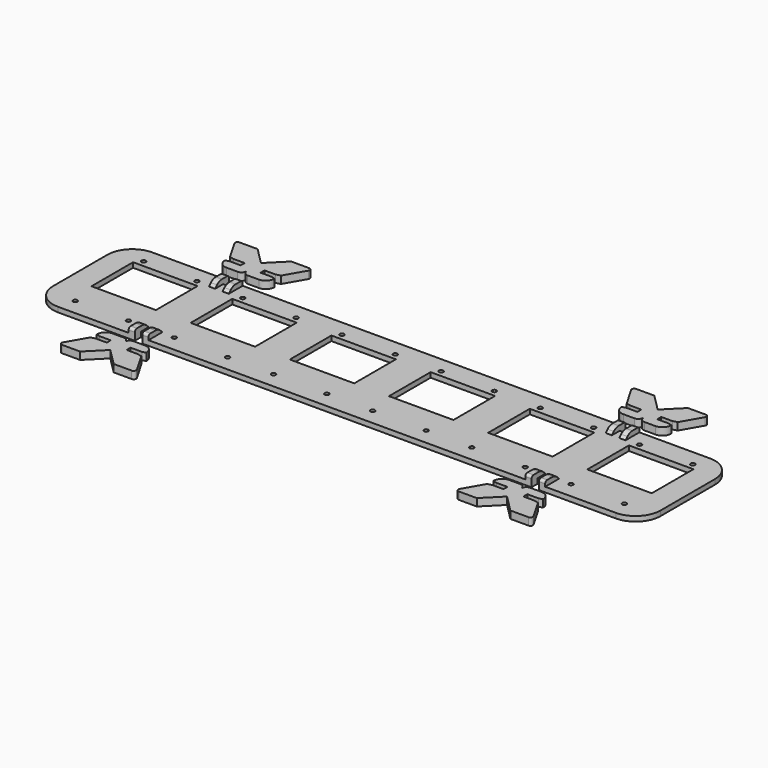
from build123d import *

# Parameters (mm, degrees)
F0_R     = 1.75
F0_W     = 52
F0_H     = 42
F1_DEPTH = 4
F2_R     = 20
F4_DEPTH = 6
F6_DEPTH = 4
F7_SIZE  = 3.99999
F8_R     = 7
F9_R     = 2


# Not quite as in the source:
# - a fillet or chamfer is up to 0.001 mm smaller than in the source, because OpenCascade refuses the exact size


with BuildPart() as f1:
    # F0 (on Top) → F1 (new body)
    with BuildSketch(Plane.XY):
        Polygon((-245, 47.5), (-245, -47.5), (-163, -47.5), (-163, -41.5), (-157, -41.5), (-157, -47.5), (157, -47.5), (157, -41.5), (163, -41.5), (163, -47.5), (245, -47.5), (245, 47.5), (163, 47.5), (163, 41.5), (157, 41.5), (157, 47.5), (-157, 47.5), (-157, 41.5), (-163, 41.5), (-163, 47.5), align=None)
        with Locations((-221.5, -34.5)):
            Circle(F0_R, mode=Mode.SUBTRACT)
        with Locations((-178.5, -34.5)):
            Circle(F0_R, mode=Mode.SUBTRACT)
        with Locations((-141.5, -34.5)):
            Circle(F0_R, mode=Mode.SUBTRACT)
        with Locations((-98.5, -34.5)):
            Circle(F0_R, mode=Mode.SUBTRACT)
        with Locations((-61.5, -34.5)):
            Circle(F0_R, mode=Mode.SUBTRACT)
        with Locations((-18.5, -34.5)):
            Circle(F0_R, mode=Mode.SUBTRACT)
        with Locations((18.5, -34.5)):
            Circle(F0_R, mode=Mode.SUBTRACT)
        with Locations((61.5, -34.5)):
            Circle(F0_R, mode=Mode.SUBTRACT)
        with Locations((98.5, -34.5)):
            Circle(F0_R, mode=Mode.SUBTRACT)
        with Locations((141.5, -34.5)):
            Circle(F0_R, mode=Mode.SUBTRACT)
        with Locations((178.5, -34.5)):
            Circle(F0_R, mode=Mode.SUBTRACT)
        with Locations((221.5, -34.5)):
            Circle(F0_R, mode=Mode.SUBTRACT)
        with Locations((-200, 8.5)):
            Rectangle(F0_W, F0_H, mode=Mode.SUBTRACT)
        with Locations((-120, 8.5)):
            Rectangle(F0_W, F0_H, mode=Mode.SUBTRACT)
        with Locations((-40, 8.5)):
            Rectangle(F0_W, F0_H, mode=Mode.SUBTRACT)
        with Locations((40, 8.5)):
            Rectangle(F0_W, F0_H, mode=Mode.SUBTRACT)
        with Locations((120, 8.5)):
            Rectangle(F0_W, F0_H, mode=Mode.SUBTRACT)
        with Locations((-221.5, 34.5)):
            Circle(F0_R, mode=Mode.SUBTRACT)
        with Locations((-178.5, 34.5)):
            Circle(F0_R, mode=Mode.SUBTRACT)
        with Locations((-141.5, 34.5)):
            Circle(F0_R, mode=Mode.SUBTRACT)
        with Locations((-98.5, 34.5)):
            Circle(F0_R, mode=Mode.SUBTRACT)
        with Locations((-61.5, 34.5)):
            Circle(F0_R, mode=Mode.SUBTRACT)
        with Locations((-18.5, 34.5)):
            Circle(F0_R, mode=Mode.SUBTRACT)
        with Locations((18.5, 34.5)):
            Circle(F0_R, mode=Mode.SUBTRACT)
        with Locations((61.5, 34.5)):
            Circle(F0_R, mode=Mode.SUBTRACT)
        with Locations((98.5, 34.5)):
            Circle(F0_R, mode=Mode.SUBTRACT)
        with Locations((141.5, 34.5)):
            Circle(F0_R, mode=Mode.SUBTRACT)
        with Locations((200, 8.5)):
            Rectangle(F0_W, F0_H, mode=Mode.SUBTRACT)
        with Locations((178.5, 34.5)):
            Circle(F0_R, mode=Mode.SUBTRACT)
        with Locations((221.5, 34.5)):
            Circle(F0_R, mode=Mode.SUBTRACT)
    extrude(amount=F1_DEPTH)

    # F2
    f2_edges = [f1.edges().sort_by_distance(p)[0] for p in [
        (-245, -47.5, 2),
        (-245, 47.5, 2),
        (245, 47.5, 2),
        (245, -47.5, 2),
    ]]
    fillet(f2_edges, radius=F2_R)

    # F5 (on face) → F6 (join)
    with BuildSketch(Plane.XY.offset(4)):
        Polygon((-168, -47.5), (-163, -47.5), (-163, -41.5), (-163, -33.5), (-168, -33.5), align=None)
        Polygon((-157, -33.5), (-157, -41.5), (-157, -47.5), (-152, -47.5), (-152, -33.5), align=None)
        Polygon((-163, 47.5), (-168, 47.5), (-168, 33.5), (-163, 33.5), (-163, 41.5), align=None)
        Polygon((-157, 47.5), (-157, 41.5), (-157, 33.5), (-152, 33.5), (-152, 47.5), align=None)
        Polygon((163, -33.5), (163, -41.5), (163, -47.5), (168, -47.5), (168, -33.5), align=None)
        Polygon((152, -33.5), (152, -47.5), (157, -47.5), (157, -41.5), (157, -33.5), align=None)
        Polygon((157, 47.5), (152, 47.5), (152, 33.5), (157, 33.5), (157, 41.5), align=None)
        Polygon((163, 47.5), (163, 41.5), (163, 33.5), (168, 33.5), (168, 47.5), align=None)
    extrude(amount=F6_DEPTH)

    # F7 (size 4 in the source; OpenCascade refuses exactly that, so slightly less here)
    f7_edges = [f1.edges().sort_by_distance(p)[0] for p in [
        (-165.5, -33.5, 8),
        (-154.5, -33.5, 8),
        (-165.5, 33.5, 8),
        (-154.5, 33.5, 8),
        (154.5, 33.5, 8),
        (165.5, 33.5, 8),
        (165.5, -33.5, 8),
        (154.5, -33.5, 8),
    ]]
    chamfer(f7_edges, length=F7_SIZE)

    # F8
    f8_edges = [f1.edges().sort_by_distance(p)[0] for p in [
        (-165.5, 37.49999, 8),
        (-154.5, 37.49999, 8),
        (-165.5, -37.49999, 8),
        (-154.5, -37.49999, 8),
        (165.5, -37.49999, 8),
        (154.5, -37.49999, 8),
        (154.5, 37.49999, 8),
        (165.5, 37.49999, 8),
    ]]
    fillet(f8_edges, radius=F8_R)

    # F9
    f9_edges = [f1.edges().sort_by_distance(p)[0] for p in [
        (-165.5, -47.5, 8),
        (-154.5, -47.5, 8),
        (-165.5, 47.5, 8),
        (-154.5, 47.5, 8),
        (165.5, -47.5, 8),
        (154.5, -47.5, 8),
        (154.5, 47.5, 8),
        (165.5, 47.5, 8),
    ]]
    fillet(f9_edges, radius=F9_R)


with BuildPart() as f4:
    # F3 (on Top) → F4 (new body)
    with BuildSketch(Plane.XY):
        with BuildLine():
            Line((-160, -75.9529946162), (-160, -61.5))
            ThreePointArc((-160, -61.5), (-161.1715728753, -58.6715728753), (-164, -57.5))
            Line((-164, -57.5), (-173, -57.5))
            ThreePointArc((-173, -57.5), (-177.9497474683, -59.5502525317), (-180, -64.5))
            Line((-180, -64.5), (-180, -64.6961524227))
            Line((-180, -64.6961524227), (-177, -65.5))
            Line((-177, -65.5), (-168, -65.5))
            Line((-168, -65.5), (-168, -69.5))
            Line((-168, -69.5), (-177, -69.5))
            Line((-177, -69.5), (-180.5490381057, -70.4509618943))
            Line((-180.5490381057, -70.4509618943), (-189.8149545762, -86.5))
            ThreePointArc((-189.8149545762, -86.5), (-189.8149545762, -88.5), (-188.0829037687, -89.5))
            Line((-188.0829037687, -89.5), (-173.5470053838, -89.5))
            Line((-173.5470053838, -89.5), (-160, -75.9529946162))
        make_face()
        with BuildLine():
            Line((-152, -69.5), (-152, -65.5))
            Line((-152, -65.5), (-143, -65.5))
            Line((-143, -65.5), (-140, -64.6961524227))
            Line((-140, -64.6961524227), (-140, -64.5))
            ThreePointArc((-140, -64.5), (-142.0502525317, -59.5502525317), (-147, -57.5))
            Line((-147, -57.5), (-156, -57.5))
            ThreePointArc((-156, -57.5), (-158.8284271247, -58.6715728753), (-160, -61.5))
            Line((-160, -61.5), (-160, -75.9529946162))
            Line((-160, -75.9529946162), (-146.4529946162, -89.5))
            Line((-146.4529946162, -89.5), (-131.9170962313, -89.5))
            ThreePointArc((-131.9170962313, -89.5), (-130.1850454238, -88.5), (-130.1850454238, -86.5))
            Line((-130.1850454238, -86.5), (-139.4509618943, -70.4509618943))
            Line((-139.4509618943, -70.4509618943), (-143, -69.5))
            Line((-143, -69.5), (-152, -69.5))
        make_face()
    extrude(amount=F4_DEPTH)


with BuildPart() as f10_1:
    # F10: instance of F4
    add(f4.part.mirror(Plane.YZ))


with BuildPart() as f11_1:
    # F11: instance of F4
    add(f4.part.mirror(Plane.XZ))


with BuildPart() as f11_2:
    # F11: instance of F10_1
    add(f10_1.part.mirror(Plane.XZ))


solid = Compound([f1.part, f4.part, f10_1.part, f11_1.part, f11_2.part])
